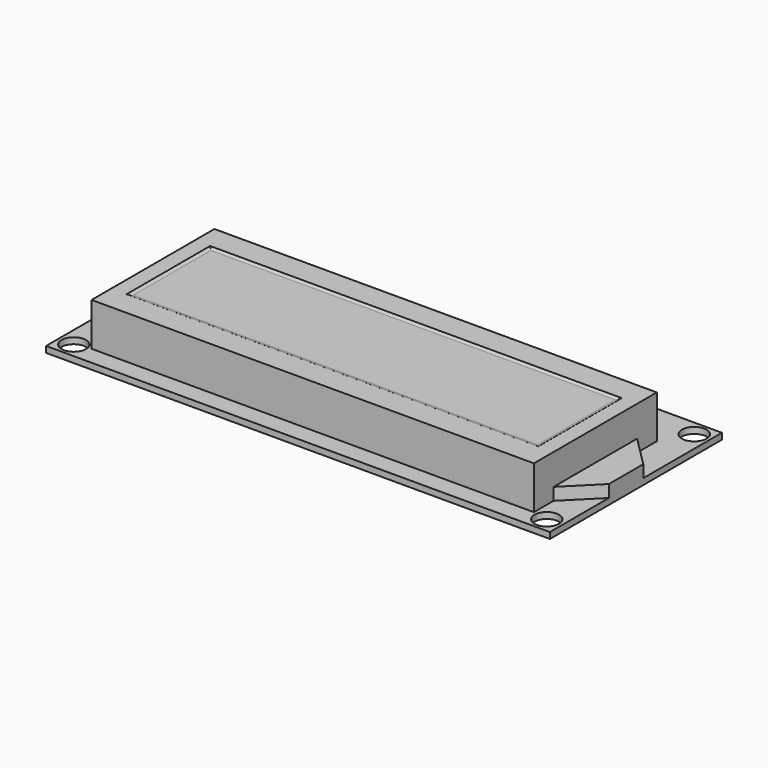
from build123d import *

# Parameters (mm, degrees)
F0_W         = 82
F0_H         = 35
F1_DEPTH     = 1
F2_W         = 72
F2_H         = 25
F3_DEPTH     = 7
F5_DEPTH     = 2
F6_R         = 2
F7_DEPTH     = 2
F8_W         = 67
F8_H         = 17
F9_DEPTH     = 0.2
F10_T1_DEPTH = 20
F10_T3_DEPTH = 70
F11_R        = 0.5
F12_DEPTH    = 2


# Not quite as in the source:
# - a fillet or chamfer that OpenCascade refuses, or shapes differently, is made with other operations: its cross-section is extruded or revolved along the edge and cut away or added


with BuildPart() as f1:
    # F0 (on Top) → F1 (new body)
    with BuildSketch(Plane.XY):
        Rectangle(F0_W, F0_H)
    extrude(amount=F1_DEPTH)

    # F2 (on face) → F3 (join)
    with BuildSketch(Plane.XY.offset(1)):
        with Locations((0, -2)):
            Rectangle(F2_W, F2_H)
    extrude(amount=F3_DEPTH)

    # F4 (on face) → F5 (join)
    with BuildSketch(Plane.XY.offset(1)):
        Polygon((36, -10.5), (41, -5.5), (41, 1.5), (36, 6.5), align=None)
    extrude(amount=F5_DEPTH)

    # F6 (on face) → F7 (cut)
    with BuildSketch(Plane.XY.offset(1)):
        with Locations((-38.5, -15)):
            Circle(F6_R)
        with Locations((38.5, -15)):
            Circle(F6_R)
        with Locations((-38.5, 15)):
            Circle(F6_R)
        with Locations((38.5, 15)):
            Circle(F6_R)
    extrude(amount=-F7_DEPTH, mode=Mode.SUBTRACT)

    # F8 (on face) → F9 (cut)
    with BuildSketch(Plane.XY.offset(8)):
        with Locations((0, -2)):
            Rectangle(F8_W, F8_H)
    extrude(amount=-F9_DEPTH, mode=Mode.SUBTRACT)

    # F10: fillet of radius 1 on 4 edges, made by hand

    # F10_s2 → F10_t1 (join)
    with BuildSketch(Plane.XZ.offset(-8)):
        with BuildLine():
            ThreePointArc((33.5, 8), (33.216227766, 7.8513167019), (32.9, 7.8))
            Line((32.9, 7.8), (33.5, 7.8))
            Line((33.5, 7.8), (33.5, 8))
        make_face()
        with BuildLine():
            ThreePointArc((-33.5, 8), (-33.216227766, 7.8513167019), (-32.9, 7.8))
            Line((-32.9, 7.8), (-33.5, 7.8))
            Line((-33.5, 7.8), (-33.5, 8))
        make_face()
    extrude(amount=F10_T1_DEPTH)

    # F10_s4 → F10_t3 (join)
    with BuildSketch(Plane.YZ.offset(-35)):
        with BuildLine():
            ThreePointArc((6.5, 8), (6.216227766, 7.8513167019), (5.9, 7.8))
            Line((5.9, 7.8), (6.5, 7.8))
            Line((6.5, 7.8), (6.5, 8))
        make_face()
        with BuildLine():
            ThreePointArc((-10.5, 8), (-10.216227766, 7.8513167019), (-9.9, 7.8))
            Line((-9.9, 7.8), (-10.5, 7.8))
            Line((-10.5, 7.8), (-10.5, 8))
        make_face()
    extrude(amount=F10_T3_DEPTH)

    # F11 (on face) → F12 (cut)
    with BuildSketch(Plane.XY.offset(1)):
        with Locations((-33.5, 15)):
            Circle(F11_R)
        with Locations((-31, 15)):
            Circle(F11_R)
        with Locations((-28.5, 15)):
            Circle(F11_R)
        with Locations((-26, 15)):
            Circle(F11_R)
        with Locations((-23.5, 15)):
            Circle(F11_R)
        with Locations((-21, 15)):
            Circle(F11_R)
        with Locations((-18.5, 15)):
            Circle(F11_R)
        with Locations((-16, 15)):
            Circle(F11_R)
        with Locations((-13.5, 15)):
            Circle(F11_R)
        with Locations((-11, 15)):
            Circle(F11_R)
        with Locations((-8.5, 15)):
            Circle(F11_R)
        with Locations((-6, 15)):
            Circle(F11_R)
        with Locations((-3.5, 15)):
            Circle(F11_R)
        with Locations((-1, 15)):
            Circle(F11_R)
        with Locations((1.5, 15)):
            Circle(F11_R)
        with Locations((4, 15)):
            Circle(F11_R)
    extrude(amount=-F12_DEPTH, mode=Mode.SUBTRACT)


solid = f1.part
